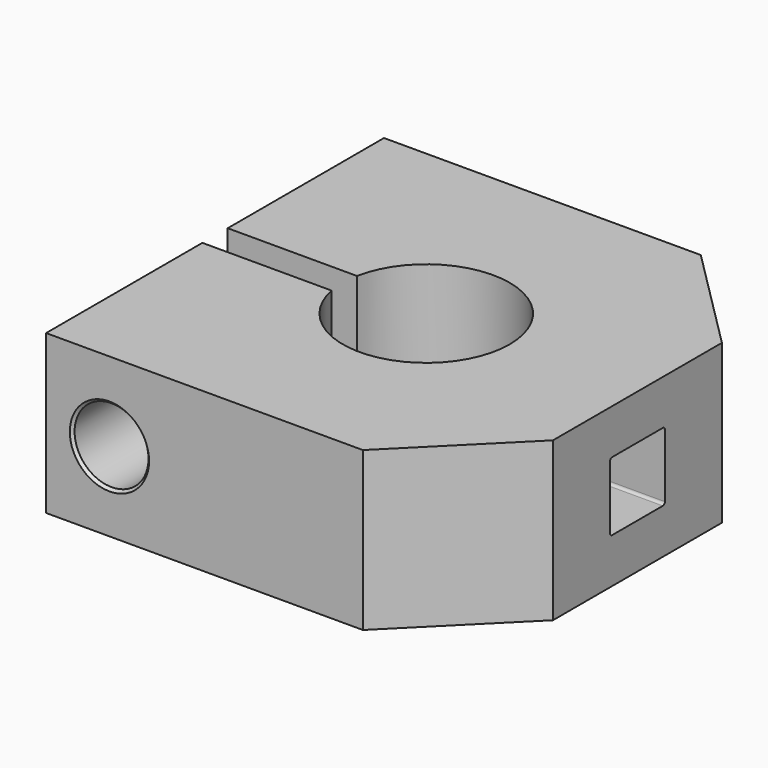
from build123d import *

# Parameters (mm, degrees)
F1_DEPTH  = 15
F2_R      = 3.5
F3_DEPTH  = 25
F5_D      = 6.6
F5_DEPTH  = 15
F5_TIP    = 1.9828400428
F6_SIZE   = 10
F7_W      = 6.5
F7_H      = 6.5
F8_DEPTH  = 12.8004791855
F10_D     = 4.4
F10_DEPTH = 5
F10_TIP   = 1.3218933619
F11_SIZE  = 0.25
F12_R     = 0.25


with BuildPart() as f1:
    # F0 (on Top) → F1 (new body)
    with BuildSketch(Plane.XY):
        with BuildLine():
            Line((20, -20), (20, 20))
            Line((20, 20), (-20, 20))
            Line((-20, 20), (-20, 1.5))
            Line((-20, 1.5), (-7.7562877719, 1.5))
            ThreePointArc((-7.7562877719, 1.5), (7.9, 0), (-7.7562877719, -1.5))
            Line((-7.7562877719, -1.5), (-20, -1.5))
            Line((-20, -1.5), (-20, -20))
            Line((-20, -20), (20, -20))
        make_face()
    extrude(amount=F1_DEPTH)

    # F2 (on Front) → F3 (cut)
    with BuildSketch(Plane.XZ):
        with Locations((-14, 7.5)):
            Circle(F2_R)
    extrude(amount=F3_DEPTH, mode=Mode.SUBTRACT)

    # F5
    with Locations(Plane.XZ.offset(-1.5)):
        with Locations((-14, 7.5)):
            Hole(F5_D / 2, depth=F5_DEPTH)
            with Locations((0, 0, -(F5_DEPTH + F5_TIP / 2))):  # 118° drill point
                Cone(0, F5_D / 2, F5_TIP, mode=Mode.SUBTRACT)

    # F6
    f6_edges = [f1.edges().sort_by_distance(p)[0] for p in [
        (20, -20, 7.5),
        (20, 20, 7.5),
    ]]
    chamfer(f6_edges, length=F6_SIZE)

    # F7 (on face) → F8 (cut, through all)
    with BuildSketch(Plane.YZ.offset(20)):
        with Locations((0, 7.5)):
            Rectangle(F7_W, F7_H)
    extrude(amount=-F8_DEPTH, mode=Mode.SUBTRACT)

    # F10
    with Locations(Plane(origin=(0, 0, 0), x_dir=(1, 0, 0), z_dir=(0, 0, -1))):
        with Locations((14, 0)):
            Hole(F10_D / 2, depth=F10_DEPTH)
            with Locations((0, 0, -(F10_DEPTH + F10_TIP / 2))):  # 118° drill point
                Cone(0, F10_D / 2, F10_TIP, mode=Mode.SUBTRACT)

    # F11
    f11_edges = [f1.edges().sort_by_distance(p)[0] for p in [
        (-17.5, -20, 7.5),
        (11.8, 0, 0),
    ]]
    chamfer(f11_edges, length=F11_SIZE)

    # F12
    f12_edges = [f1.edges().sort_by_distance(p)[0] for p in [
        (13.60026, 3.25, 4.25),
        (13.60026, -3.25, 4.25),
        (13.60026, 3.25, 10.75),
        (13.60026, -3.25, 10.75),
    ]]
    fillet(f12_edges, radius=F12_R)


solid = f1.part
